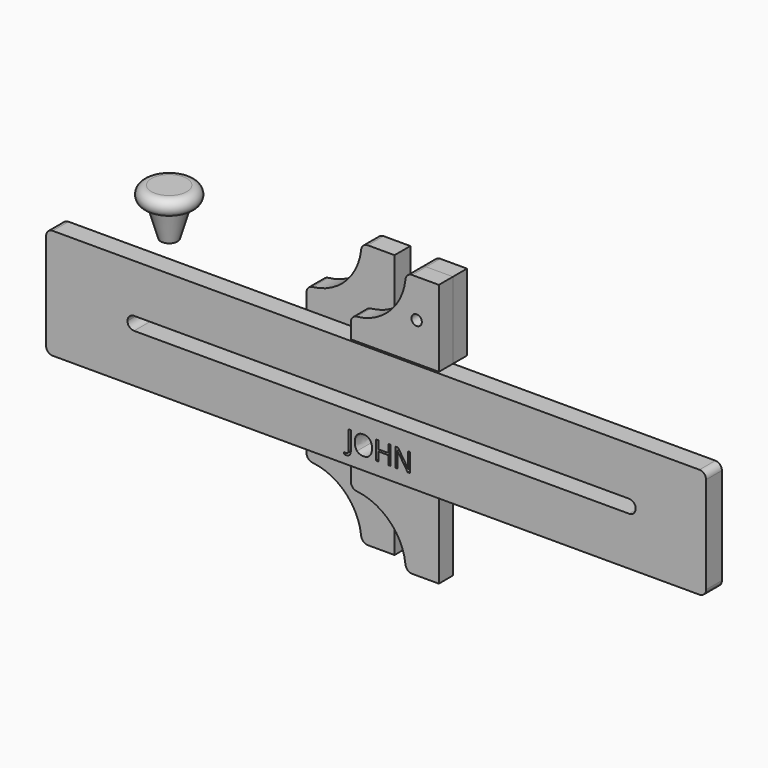
from build123d import *

# Parameters (mm, degrees)
F1_DEPTH = 18
F3_DEPTH = 18
F5_R     = 4.7266267097
F6_DEPTH = 16


# Not quite as in the source:
# - the program builds the solid bodies; features that only make, move or delete a surface that nothing else refers to are left out


with BuildPart() as f1:
    # F0 (on Front) → F1 (new body)
    with BuildSketch(Plane.XZ):
        with BuildLine():
            Line((291.639387846, 50.4278332508), (-296.360612154, 50.4278332508))
            ThreePointArc((-296.360612154, 50.4278332508), (-300.6032528411, 48.6704739379), (-302.360612154, 44.4278332508))
            Line((-302.360612154, 44.4278332508), (-302.360612154, 0.4278332508))
            Line((-302.360612154, 0.4278332508), (-228.3910287511, 0.4278332508))
            ThreePointArc((-228.3910287511, 0.4278332508), (-226.6320094967, 4.6744441775), (-222.3853767709, 6.4334108038))
            Line((-222.3853767709, 6.4334108038), (227.6739476629, 6.4278332503))
            ThreePointArc((227.6739476629, 6.4278332503), (231.9165402817, 4.6704476485), (233.6738733053, 0.4278332508))
            Line((233.6738733053, 0.4278332508), (297.639387846, 0.4278332508))
            Line((297.639387846, 0.4278332508), (297.639387846, 44.4278332508))
            ThreePointArc((297.639387846, 44.4278332508), (295.8820285331, 48.6704739379), (291.639387846, 50.4278332508))
        make_face()
        with BuildLine():
            Line((-228.3910287511, 0.4278332508), (-302.360612154, 0.4278332508))
            Line((-302.360612154, 0.4278332508), (-302.360612154, -43.5721667492))
            ThreePointArc((-302.360612154, -43.5721667492), (-300.6032528411, -47.8148074363), (-296.360612154, -49.5721667492))
            Line((-296.360612154, -49.5721667492), (291.639387846, -49.5721667492))
            ThreePointArc((291.639387846, -49.5721667492), (295.8820285331, -47.8148074363), (297.639387846, -43.5721667492))
            Line((297.639387846, -43.5721667492), (297.639387846, 0.4278332508))
            Line((297.639387846, 0.4278332508), (233.6738733053, 0.4278332508))
            ThreePointArc((233.6738733053, 0.4278332508), (231.9165402817, -3.8147811469), (227.6739476629, -5.5721667487))
            Line((227.6739476629, -5.5721667487), (-222.3853767709, -5.5777443022))
            ThreePointArc((-222.3853767709, -5.5777443022), (-226.6320094967, -3.8187776759), (-228.3910287511, 0.4278332508))
        make_face()
        with BuildLine():
            add(Edge.make_bspline(
                [(-26.460121604, -41.1747165951), (-27.5783300604, -42.3917001317), (-29.6768345967, -42.3917001317)],
                knots=[0, 0, 0, 1, 1, 1], degree=2))
            add(Edge.make_bspline(
                [(-29.6768345967, -42.3917001317), (-30.7689515224, -42.3917001317), (-31.3988756194, -42.0786017639)],
                knots=[0, 0, 0, 1, 1, 1], degree=2))
            Line((-31.3988756194, -42.0786017639), (-31.3988756194, -40.3901069949))
            add(Edge.make_bspline(
                [(-31.3988756194, -40.3901069949), (-30.5714013618, -40.6212034092), (-29.6768345967, -40.6212034092)],
                knots=[0, 0, 0, 1, 1, 1], degree=2))
            add(Edge.make_bspline(
                [(-29.6768345967, -40.6212034092), (-28.5213525252, -40.6212034092), (-27.9212473203, -39.922323124)],
                knots=[0, 0, 0, 1, 1, 1], degree=2))
            add(Edge.make_bspline(
                [(-27.9212473203, -39.922323124), (-27.3211421154, -39.2234428388), (-27.3211421154, -37.9076842219)],
                knots=[0, 0, 0, 1, 1, 1], degree=2))
            Line((-27.3211421154, -37.9076842219), (-27.3211421154, -20.8773694321))
            Line((-27.3211421154, -20.8773694321), (-25.3419131477, -20.8773694321))
            Line((-25.3419131477, -20.8773694321), (-25.3419131477, -37.7436803149))
            add(Edge.make_bspline(
                [(-25.3419131477, -37.7436803149), (-25.3419131477, -39.9577330584), (-26.460121604, -41.1747165951)],
                knots=[0, 0, 0, 1, 1, 1], degree=2))
        make_face(mode=Mode.SUBTRACT)
        with BuildLine():
            add(Edge.make_bspline(
                [(-8.1028661128, -22.9386003533), (-6.0416351917, -25.2682013039), (-6.0416351917, -29.3682989771)],
                knots=[0, 0, 0, 1, 1, 1], degree=2))
            add(Edge.make_bspline(
                [(-6.0416351917, -29.3682989771), (-6.0416351917, -33.4572145657), (-8.1103208358, -35.7998612817)],
                knots=[0, 0, 0, 1, 1, 1], degree=2))
            add(Edge.make_bspline(
                [(-8.1103208358, -35.7998612817), (-10.17900648, -38.1425079977), (-13.8579123013, -38.1425079977)],
                knots=[0, 0, 0, 1, 1, 1], degree=2))
            add(Edge.make_bspline(
                [(-13.8579123013, -38.1425079977), (-17.6188200761, -38.1425079977), (-19.6632778704, -35.8408622584)],
                knots=[0, 0, 0, 1, 1, 1], degree=2))
            add(Edge.make_bspline(
                [(-19.6632778704, -35.8408622584), (-21.7077356647, -33.5392165192), (-21.7077356647, -29.345934808)],
                knots=[0, 0, 0, 1, 1, 1], degree=2))
            add(Edge.make_bspline(
                [(-21.7077356647, -29.345934808), (-21.7077356647, -25.1861993505), (-19.6576868281, -22.8975993765)],
                knots=[0, 0, 0, 1, 1, 1], degree=2))
            add(Edge.make_bspline(
                [(-19.6576868281, -22.8975993765), (-17.6076379915, -20.6089994026), (-13.8355481322, -20.6089994026)],
                knots=[0, 0, 0, 1, 1, 1], degree=2))
            add(Edge.make_bspline(
                [(-13.8355481322, -20.6089994026), (-10.1640970339, -20.6089994026), (-8.1028661128, -22.9386003533)],
                knots=[0, 0, 0, 1, 1, 1], degree=2))
        make_face(mode=Mode.SUBTRACT)
        Polygon((10.6830359534, -20.8773694321), (10.6830359534, -37.9076842219), (8.7038069857, -37.9076842219), (8.7038069857, -29.8938569516), (-0.2679521955, -29.8938569516), (-0.2679521955, -37.9076842219), (-2.2471811632, -37.9076842219), (-2.2471811632, -20.8773694321), (-0.2679521955, -20.8773694321), (-0.2679521955, -28.1233602291), (8.7038069857, -28.1233602291), (8.7038069857, -20.8773694321), align=None, mode=Mode.SUBTRACT)
        with BuildLine():
            Line((28.6563732079, -20.8773694321), (28.6563732079, -37.9076842219))
            Line((28.6563732079, -37.9076842219), (26.3975921262, -37.9076842219))
            Line((26.3975921262, -37.9076842219), (17.0903704081, -23.6169801501))
            Line((17.0903704081, -23.6169801501), (16.99718637, -23.6169801501))
            add(Edge.make_bspline(
                [(16.99718637, -23.6169801501), (17.1835544461, -26.1329491768), (17.1835544461, -28.2277263517)],
                knots=[0, 0, 0, 1, 1, 1], degree=2))
            Line((17.1835544461, -28.2277263517), (17.1835544461, -37.9076842219))
            Line((17.1835544461, -37.9076842219), (15.3534199393, -37.9076842219))
            Line((15.3534199393, -37.9076842219), (15.3534199393, -20.8773694321))
            Line((15.3534199393, -20.8773694321), (17.5898368519, -20.8773694321))
            Line((17.5898368519, -20.8773694321), (26.8746944009, -35.1121630811))
            Line((26.8746944009, -35.1121630811), (26.9678784389, -35.1121630811))
            add(Edge.make_bspline(
                [(26.9678784389, -35.1121630811), (26.9455142698, -34.7990647133), (26.8635123163, -33.0919331367)],
                knots=[0, 0, 0, 1, 1, 1], degree=2))
            add(Edge.make_bspline(
                [(26.8635123163, -33.0919331367), (26.7815103628, -31.38480156), (26.803874532, -30.6505113404)],
                knots=[0, 0, 0, 1, 1, 1], degree=2))
            Line((26.803874532, -30.6505113404), (26.803874532, -20.8773694321))
            Line((26.803874532, -20.8773694321), (28.6563732079, -20.8773694321))
        make_face(mode=Mode.SUBTRACT)
    extrude(amount=F1_DEPTH)


with BuildPart() as f3:
    # F2 (on Front) → F3 (new body)
    with BuildSketch(Plane.XZ):
        with BuildLine():
            Line((0, 0), (0, 120))
            Line((0, 120), (-24.3223563717, 120))
            ThreePointArc((-24.3223563717, 120), (-28.3312750004, 118.4641428549), (-30.287818189, 114.6428571429))
            ThreePointArc((-30.287818189, 114.6428571429), (-44.6446609407, 84.6446609407), (-74.6428571429, 70.287818189))
            ThreePointArc((-74.6428571429, 70.287818189), (-78.4641428549, 68.3312750004), (-80, 64.3223563717))
            Line((-80, 64.3223563717), (-80, 6))
            Line((-80, 6), (-80, 0))
            Line((-80, 0), (-48.5, 0))
            ThreePointArc((-48.5, 0), (-40, 8.5), (-31.5, 0))
            Line((-31.5, 0), (0, 0))
        make_face()
        with BuildLine():
            Line((0, -120), (0, 0))
            Line((0, 0), (-31.5, 0))
            ThreePointArc((-31.5, 0), (-40, -8.5), (-48.5, 0))
            Line((-48.5, 0), (-80, 0))
            Line((-80, 0), (-80, -6))
            Line((-80, -6), (-80, -64.3223563717))
            ThreePointArc((-80, -64.3223563717), (-78.4641428549, -68.3312750004), (-74.6428571429, -70.287818189))
            ThreePointArc((-74.6428571429, -70.287818189), (-44.6446609407, -84.6446609407), (-30.287818189, -114.6428571429))
            ThreePointArc((-30.287818189, -114.6428571429), (-28.3312750004, -118.4641428549), (-24.3223563717, -120))
            Line((-24.3223563717, -120), (0, -120))
        make_face()
    extrude(amount=-F3_DEPTH)


with BuildPart() as f6:
    # F5 (on Front) → F6 (new body)
    with BuildSketch(Plane.XZ):
        with BuildLine():
            ThreePointArc((28.7686937244, 120), (24.7597750957, 118.4641428549), (22.8032319071, 114.6428571429))
            ThreePointArc((22.8032319071, 114.6428571429), (8.4463891554, 84.6446609407), (-21.5518070468, 70.287818189))
            ThreePointArc((-21.5518070468, 70.287818189), (-25.3730533867, 68.3313188428), (-26.9089499028, 64.3224742245))
            Line((-26.9089499028, 64.3224742245), (-26.9092228264, 50.4276715219))
            Line((-26.9092228264, 50.4276715219), (53.1530342776, 50.4260989282))
            Line((53.1530342776, 50.4260989282), (53.0910500961, 120))
            Line((53.0910500961, 120), (28.7686937244, 120))
        make_face()
        with Locations((32.9252704978, 85.2130494641)):
            Circle(F5_R, mode=Mode.SUBTRACT)
    extrude(amount=F6_DEPTH)


with BuildPart() as f6b:
    # F5 (on Front) → F6, piece 2 (new body)
    with BuildSketch(Plane.XZ):
        with BuildLine():
            Line((53.0910500961, -119.1443334984), (53.1530342776, -49.5704324266))
            Line((53.1530342776, -49.5704324266), (-26.9092228264, -49.5720050203))
            Line((-26.9092228264, -49.5720050203), (-26.9089499028, -63.4668077229))
            ThreePointArc((-26.9089499028, -63.4668077229), (-25.3730533867, -67.4756523413), (-21.5518070468, -69.4321516874))
            ThreePointArc((-21.5518070468, -69.4321516874), (8.4463891554, -83.7889944391), (22.8032319071, -113.7871906413))
            ThreePointArc((22.8032319071, -113.7871906413), (24.7597750957, -117.6084763533), (28.7686937244, -119.1443334984))
            Line((28.7686937244, -119.1443334984), (53.0910500961, -119.1443334984))
        make_face()
    extrude(amount=F6_DEPTH)


with BuildPart() as f8:
    # F7 (on face) → F8 (revolve)
    with BuildSketch(Plane.XZ.offset(18)):
        with BuildLine():
            Line((-190.4600858688, 106.5727323294), (-190.4600858688, 78.7520706654))
            Line((-190.4600858688, 78.7520706654), (-182.8263103962, 78.7520706654))
            Line((-182.8263103962, 78.7520706654), (-174.5630651712, 106.5727323294))
            ThreePointArc((-174.5630651712, 106.5727323294), (-166.1744728131, 113.899124468), (-174.3393093348, 121.4740797877))
            Line((-174.3393093348, 121.4740797877), (-190.4600858688, 121.4740797877))
            Line((-190.4600858688, 121.4740797877), (-190.4600858688, 106.5727323294))
        make_face()
    revolve(axis=Axis((-190.4600858688, -18, 92.6624014974), (0, 0, 1)))


with BuildPart() as f9_1:
    # F9: instance of F6
    add(f6.part.mirror(Plane.XZ))


solid = Compound([f1.part, f3.part, f6.part, f6b.part, f8.part, f9_1.part])
